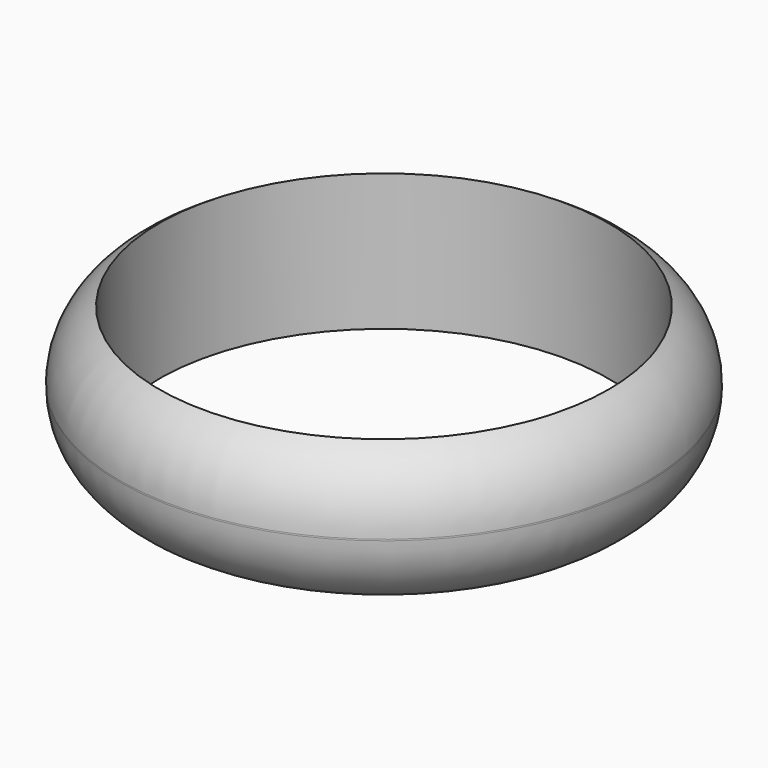
from build123d import *

# Parameters (mm, degrees)
F1_DEPTH = 7


# Not quite as in the source:
# - a fillet or chamfer that OpenCascade refuses, or shapes differently, is made with other operations: its cross-section is extruded or revolved along the edge and cut away or added


with BuildPart() as f1:
    # F0 (on Top) → F1 (new body)
    with BuildSketch(Plane.XY):
        with BuildLine():
            add(Edge.make_bspline(
                [(13.1976233846, 2.8412562359), (12.7543193448, 2.998887413), (12.1645348864, 2.998887413)],
                knots=[0.5436658964, 0.5436658964, 0.5436658964, 1, 1, 1], degree=2))
            ThreePointArc((13.1976233846, 2.8412562359), (13.0637191054, 3.4042977449), (12.9058058181, 3.9610827038))
            add(Edge.make_bspline(
                [(12.018496466, 4.0576659611), (12.4931073142, 4.0576659611), (12.9058058181, 3.9610827038)],
                knots=[0, 0, 0, 0.2797621817, 0.2797621817, 0.2797621817], degree=2))
            add(Edge.make_bspline(
                [(10.827785056, 3.8741542019), (11.3656221499, 4.0576659611), (12.018496466, 4.0576659611)],
                knots=[0.5990524264, 0.5990524264, 0.5990524264, 1, 1, 1], degree=2))
            ThreePointArc((10.827785056, 3.8741542019), (11.0081830755, 3.3271467319), (11.1609661112, 2.7717928251))
            add(Edge.make_bspline(
                [(12.1645348864, 2.998887413), (11.5938854263, 2.998887413), (11.1609661112, 2.7717928251)],
                knots=[0, 0, 0, 0.5130235885, 0.5130235885, 0.5130235885], degree=2))
        make_face()
        with BuildLine():
            add(Edge.make_bspline(
                [(12.018496466, 4.0576659611), (12.4931073142, 4.0576659611), (12.9058058181, 3.9610827038)],
                knots=[0, 0, 0, 0.2797621817, 0.2797621817, 0.2797621817], degree=2))
            ThreePointArc((12.9058058181, 3.9610827038), (-13.4966928875, 0.298799434), (12.7178605176, -4.5283577438))
            add(Edge.make_bspline(
                [(12.7178605176, -4.5283577438), (12.3876756196, -4.5853745545), (12.018496466, -4.5853745545)],
                knots=[0.7881598521, 0.7881598521, 0.7881598521, 1, 1, 1], degree=2))
            add(Edge.make_bspline(
                [(12.018496466, -4.5853745545), (11.2545246965, -4.5853745545), (10.6490584992, -4.3413768647)],
                knots=[0, 0, 0, 0.4670809567, 0.4670809567, 0.4670809567], degree=2))
            ThreePointArc((10.6490584992, -4.3413768647), (-11.4972796761, 0.2501200705), (10.827785056, 3.8741542019))
            add(Edge.make_bspline(
                [(10.827785056, 3.8741542019), (11.3656221499, 4.0576659611), (12.018496466, 4.0576659611)],
                knots=[0.5990524264, 0.5990524264, 0.5990524264, 1, 1, 1], degree=2))
        make_face()
        with BuildLine():
            ThreePointArc((12.7178605176, -4.5283577438), (12.8998623637, -3.9803958343), (13.0582667038, -3.4251526523))
            add(Edge.make_bspline(
                [(12.1791387284, -3.5265960064), (12.6699509158, -3.5265960064), (13.0582667038, -3.4251526523)],
                knots=[0, 0, 0, 0.3797562591, 0.3797562591, 0.3797562591], degree=2))
            add(Edge.make_bspline(
                [(11.0330024584, -3.2438953054), (11.5107805963, -3.5265960064), (12.1791387284, -3.5265960064)],
                knots=[0.410739346, 0.410739346, 0.410739346, 1, 1, 1], degree=2))
            ThreePointArc((11.0330024584, -3.2438953054), (10.8549094094, -3.7974915029), (10.6490584992, -4.3413768647))
            add(Edge.make_bspline(
                [(12.018496466, -4.5853745545), (11.2545246965, -4.5853745545), (10.6490584992, -4.3413768647)],
                knots=[0, 0, 0, 0.4670809567, 0.4670809567, 0.4670809567], degree=2))
            add(Edge.make_bspline(
                [(12.7178605176, -4.5283577438), (12.3876756196, -4.5853745545), (12.018496466, -4.5853745545)],
                knots=[0.7881598521, 0.7881598521, 0.7881598521, 1, 1, 1], degree=2))
        make_face()
        with BuildLine():
            ThreePointArc((13.0582667038, -3.4251526523), (13.3891112569, -1.7267598991), (13.5, 0))
            ThreePointArc((13.5, 0), (13.4241930054, 1.428650466), (13.1976233846, 2.8412562359))
            add(Edge.make_bspline(
                [(13.1976233846, 2.8412562359), (12.7543193448, 2.998887413), (12.1645348864, 2.998887413)],
                knots=[0.5436658964, 0.5436658964, 0.5436658964, 1, 1, 1], degree=2))
            add(Edge.make_bspline(
                [(12.1645348864, 2.998887413), (11.5938854263, 2.998887413), (11.1609661112, 2.7717928251)],
                knots=[0, 0, 0, 0.5130235885, 0.5130235885, 0.5130235885], degree=2))
            ThreePointArc((11.1609661112, 2.7717928251), (11.4149268565, 1.3962252185), (11.5, 0))
            ThreePointArc((11.5, 0), (11.3826518938, -1.6386689306), (11.0330024584, -3.2438953054))
            add(Edge.make_bspline(
                [(11.0330024584, -3.2438953054), (11.5107805963, -3.5265960064), (12.1791387284, -3.5265960064)],
                knots=[0.410739346, 0.410739346, 0.410739346, 1, 1, 1], degree=2))
            add(Edge.make_bspline(
                [(12.1791387284, -3.5265960064), (12.6699509158, -3.5265960064), (13.0582667038, -3.4251526523)],
                knots=[0, 0, 0, 0.3797562591, 0.3797562591, 0.3797562591], degree=2))
        make_face()
    extrude(amount=F1_DEPTH)

    # F2: fillet of radius 4 on 1 edges, made by hand

    # F2_s1 → F2_t2 (revolve, cut)
    with BuildSketch(Plane(origin=(0, 0, 0), x_dir=(0, 0, 1), z_dir=(-0.2537150113, -0.9672790151, 0))):
        with BuildLine():
            ThreePointArc((3.5358983849, -13.5), (5.5358983849, -12.9641016151), (7, -11.5))
            Line((7, -11.5), (7, -13.5))
            Line((7, -13.5), (3.5358983849, -13.5))
        make_face()
    revolve(axis=Axis((0, 0, 7), (0, 0, 1)), mode=Mode.SUBTRACT)

    # F3: fillet of radius 4 on 1 edges, made by hand

    # F3_s1 → F3_t2 (revolve, cut)
    with BuildSketch(Plane(origin=(0, 0, 0), x_dir=(0, 0, 1), z_dir=(-0.2537150113, -0.9672790151, 0))):
        with BuildLine():
            ThreePointArc((0, -11.5), (1.4641016151, -12.9641016151), (3.4641016151, -13.5))
            Line((3.4641016151, -13.5), (0, -13.5))
            Line((0, -13.5), (0, -11.5))
        make_face()
    revolve(axis=Axis((0, 0, 0), (0, 0, 1)), mode=Mode.SUBTRACT)


solid = f1.part
